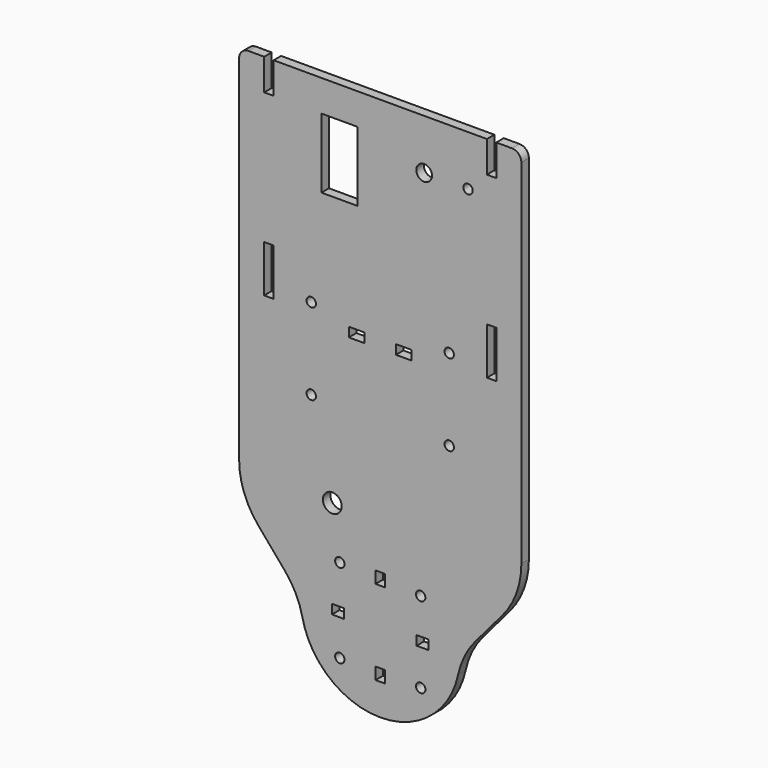
from build123d import *

# Parameters (mm, degrees)
F0_W      = 90
F0_H      = 125
F1_DEPTH  = 3
F3_R      = 2.5
F3_R_2    = 1.5
F4_DEPTH  = 25.4
F5_R      = 25.4
F2_W      = 3
F2_H      = 5
F2_H_2    = 15
F2_H_3    = 10
F2_W_2    = 5
F2_H_4    = 3
F6_DEPTH  = 25.4
F7_W      = 3.81
F7_H      = 1.5
F7_W_2    = 1.5
F7_H_2    = 3.81
F7_R      = 1.5
F8_DEPTH  = 25.4
F9_R      = 3
F11_DEPTH = 25.4
F12_R     = 25.4
F13_R     = 1.5
F14_DEPTH = 3
F16_DEPTH = 3


# Not quite as in the source:
# - a feature names something its author has since deleted; it is built from what else it names


with BuildPart() as f1:
    # F0 (on Front) → F1 (new body)
    with BuildSketch(Plane.XZ):
        with Locations((-45, 62.5)):
            Rectangle(F0_W, F0_H)
        Polygon((-45, -70), (0, 0), (-90, 0), align=None)
    extrude(amount=F1_DEPTH)

    # F3 (on face) → F4 (cut)
    with BuildSketch(Plane.XZ.offset(3)):
        Polygon((-59, 115), (-63.75, 115), (-63.75, 109), (-58, 109), (-58, 115), align=None)
        Polygon((-58, 109), (-63.75, 109), (-63.75, 92.8), (-59, 92.8), (-58, 92.8), align=None)
        Polygon((-57, 115), (-58, 115), (-58, 109), (-52.25, 109), (-52.25, 115), align=None)
        Polygon((-52.25, 109), (-58, 109), (-58, 92.8), (-57, 92.8), (-52.25, 92.8), align=None)
        with Locations((-31, 109)):
            Circle(F3_R)
        with Locations((-17, 109)):
            Circle(F3_R_2)
    extrude(amount=-F4_DEPTH, mode=Mode.SUBTRACT)

    # F5
    f5_edges = [f1.edges().sort_by_distance(p)[0] for p in [
        (-45, -1.5, -70),
    ]]
    fillet(f5_edges, radius=F5_R)

    # F2 (on face) → F6 (cut)
    with BuildSketch(Plane.XZ.offset(3)):
        with Locations((-80.5, 127.5)):
            Rectangle(F2_W, F2_H)
        with Locations((-9.5, 127.5)):
            Rectangle(F2_W, F2_H)
        with Locations((-9.5, 65.5)):
            Rectangle(F2_W, F2_H_2)
        with Locations((-80.5, 65.5)):
            Rectangle(F2_W, F2_H_2)
        with Locations((-80.5, 120)):
            Rectangle(F2_W, F2_H_3)
        with Locations((-9.5, 120)):
            Rectangle(F2_W, F2_H_3)
        with Locations((-52.5, 56.5)):
            Rectangle(F2_W_2, F2_H_4)
        with Locations((-37.5, 56.5)):
            Rectangle(F2_W_2, F2_H_4)
    extrude(amount=-F6_DEPTH, mode=Mode.SUBTRACT)

    # F7 (on face) → F8 (cut)
    with BuildSketch(Plane.XZ.offset(3)):
        with Locations((-58.495, -22.2788609758)):
            Rectangle(F7_W, F7_H)
        with Locations((-58.495, -23.7788609758)):
            Rectangle(F7_W, F7_H)
        with Locations((-31.505, -22.2788609758)):
            Rectangle(F7_W, F7_H)
        with Locations((-31.505, -23.7788609758)):
            Rectangle(F7_W, F7_H)
        with Locations((-44.25, -36.5238609758)):
            Rectangle(F7_W_2, F7_H_2)
        with Locations((-45.75, -36.5238609758)):
            Rectangle(F7_W_2, F7_H_2)
        with Locations((-44.25, -9.5338609758)):
            Rectangle(F7_W_2, F7_H_2)
        with Locations((-45.75, -9.5338609758)):
            Rectangle(F7_W_2, F7_H_2)
        with Locations((-57.9, -9.1288609758)):
            Circle(F7_R)
        with Locations((-32.1, -10.1288609758)):
            Circle(F7_R)
        with Locations((-32.1, -35.9288609758)):
            Circle(F7_R)
        with Locations((-57.9, -35.9288609758)):
            Circle(F7_R)
    extrude(amount=-F8_DEPTH, mode=Mode.SUBTRACT)

    # F9
    f9_edges = [f1.edges().sort_by_distance(p)[0] for p in [
        (0, -1.5, 125),
        (-90, -1.5, 125),
    ]]
    fillet(f9_edges, radius=F9_R)

    # F10 (on face) → F11 (cut)
    with BuildSketch(Plane.XZ.offset(3)):
        with BuildLine():
            ThreePointArc((-66.3659332746, -36.7641037951), (-69.3706247886, -30.1865594475), (-70.4, -23.0288609758))
            Line((-70.4, -23.0288609758), (-90, 0))
            Line((-90, 0), (-66.3659332746, -36.7641037951))
        make_face()
        with BuildLine():
            Line((0, 0), (-19.6, -23.0288609758))
            ThreePointArc((-19.6, -23.0288609758), (-20.6293752114, -30.1865594475), (-23.6340667254, -36.7641037951))
            Line((-23.6340667254, -36.7641037951), (0, 0))
        make_face()
    extrude(amount=-F11_DEPTH, mode=Mode.SUBTRACT)

    # F12
    f12_edges = [f1.edges().sort_by_distance(p)[0] for p in [
        (-70.4, -1.5, -23.028861),
        (-90, -1.5, 0),
        (-19.6, -1.5, -23.028861),
        (0, -1.5, 0),
    ]]
    fillet(f12_edges, radius=F12_R)

    # F13 (on face) → F14 (cut, through all)
    with BuildSketch(Plane(origin=(0, 0, 0), x_dir=(-1, 0, 0), z_dir=(0, 1, 0))):
        with Locations((23, 61)):
            Circle(F13_R)
        with Locations((23, 35)):
            Circle(F13_R)
        with Locations((67, 35)):
            Circle(F13_R)
        with Locations((67, 61)):
            Circle(F13_R)
    extrude(amount=-F14_DEPTH, mode=Mode.SUBTRACT)

    # F15 (on face) → F16 (cut)
    with BuildSketch(Plane.XZ.offset(3)):
        with BuildLine():
            ThreePointArc((-57.2929937846, 6.804616942), (-60.2929937846, 9.804616942), (-63.2929937846, 6.804616942))
            ThreePointArc((-63.2929937846, 6.804616942), (-60.2929937846, 3.804616942), (-57.2929937846, 6.804616942))
        make_face()
    extrude(amount=-F16_DEPTH, mode=Mode.SUBTRACT)


solid = f1.part
